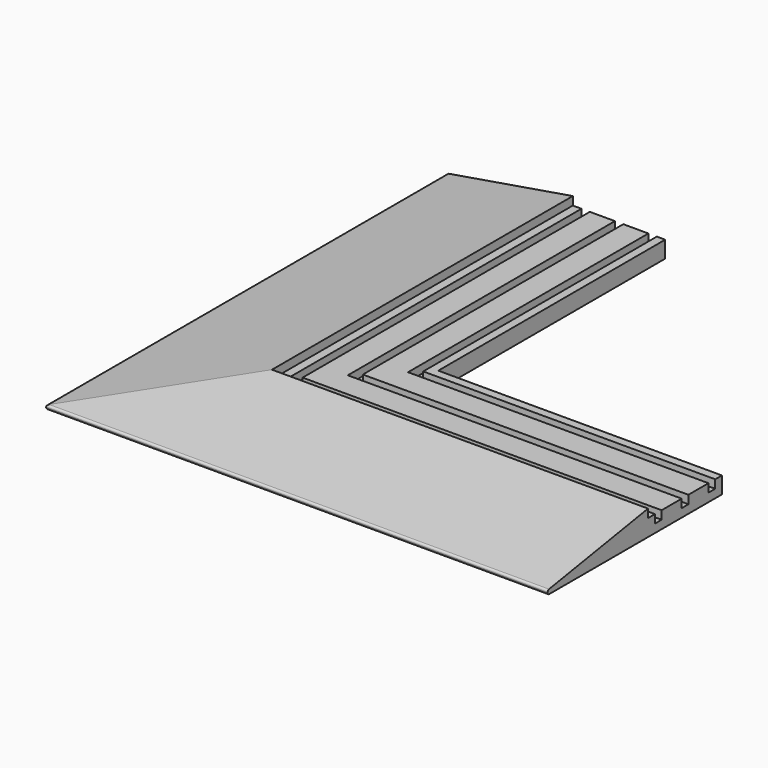
from build123d import *

# Parameters (mm, degrees)
F0_W        = 30
F0_H        = 10
F0_W_2      = 10.3326633751
F1_DEPTH    = 600
F2_T1_DEPTH = 1362.4185197182
F3_SIZE2    = 149.99999
F3_SIZE     = 24.99999
F4_R        = 2.5


# Not quite as in the source:
# - a fillet or chamfer that OpenCascade refuses, or shapes differently, is made with other operations: its cross-section is extruded or revolved along the edge and cut away or added
# - a fillet or chamfer is up to 0.001 mm smaller than in the source, because OpenCascade refuses the exact size


with BuildPart() as f1:
    # F0 (on Front) → F1 (new body)
    with BuildSketch(Plane.XZ):
        Polygon((0, -10), (0, 0), (-150, 0), (-150, -30), (0, -30), (0, -20), align=None)
        with Locations((75.3326633751, -15)):
            Rectangle(F0_W, F0_H)
        with Locations((5.1663316875, -15)):
            Rectangle(F0_W_2, F0_H)
        with Locations((35.3326633751, -15)):
            Rectangle(F0_W, F0_H)
        Polygon((10.3326633751, -20), (0, -20), (0, -30), (100.4177228767, -30), (100.4177228767, -20), (90.3326633751, -20), (60.3326633751, -20), (50.3326633751, -20), (20.3326633751, -20), align=None)
        Polygon((100.4177228767, -20), (100.4177228767, -30), (110.4177228767, -30), (110.4177228767, -10), (100.4177228767, -10), align=None)
    extrude(amount=F1_DEPTH)

    # F2: chamfer of 261 on 1 edges, made by hand

    # F2_s2 → F2_t1 (cut)
    with BuildSketch(Plane.XY.offset(-701.2092598591)):
        Polygon((110.4177228767, -339), (-150.5822771233, -600), (110.4177228767, -600), align=None)
    extrude(amount=F2_T1_DEPTH, mode=Mode.SUBTRACT)

    # F3 (size 25 and 150 in the source; OpenCascade refuses exactly that, so slightly less here)
    f3_edges = [f1.edges().sort_by_distance(p)[0] for p in [
        (-150, -299.708861, 0),
    ]]
    f3_side = f1.faces().sort_by_distance((-150, -299.708861, -15))[0]
    chamfer(f3_edges, length=F3_SIZE, length2=F3_SIZE2, reference=f3_side)

    # F4
    f4_edges = [f1.edges().sort_by_distance(p)[0] for p in [
        (-150, -299.708861, -24.99999),
        (-150, -299.708861, -30),
    ]]
    fillet(f4_edges, radius=F4_R)

    # F5: F1 across face


with BuildPart() as f1_1:
    add(f1.part)
    add(f1.part.mirror(Plane(origin=(-9.807206416, -459.2249292927, -20.1902158269), x_dir=(0.7071067812, 0.7071067812, 0), z_dir=(0.7071067812, -0.7071067812, 0))))


solid = f1_1.part
